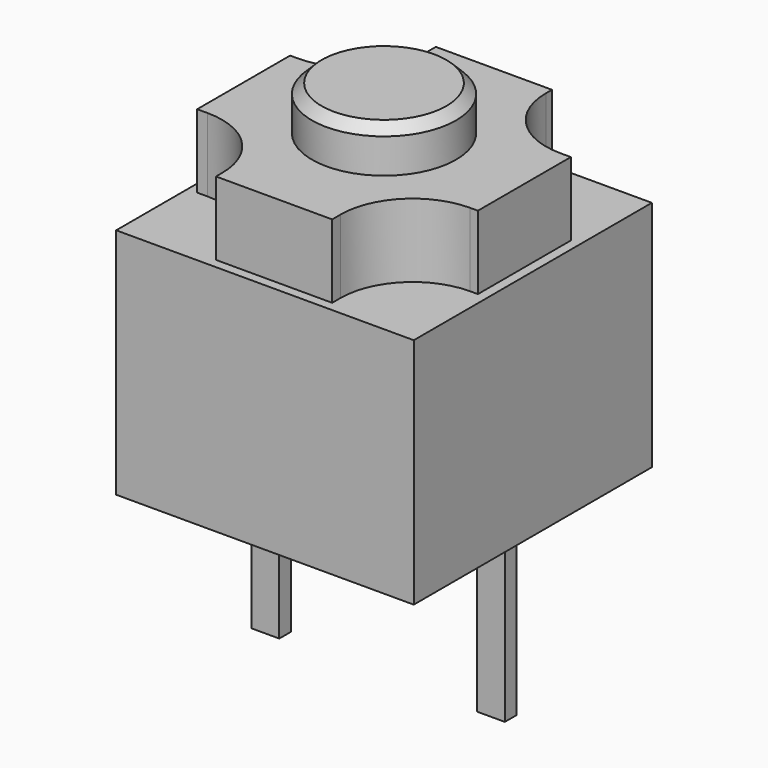
from build123d import *

# Parameters (mm, degrees)
F0_W            = 6.2
F0_H            = 6.2
F1_DEPTH        = 4.85
F3_DEPTH        = 1.53
F3_COPIES_COUNT = 4
F5_R            = 1.5
F6_DEPTH        = 0.92
F7_SIZE         = 0.2
F8_W            = 0.5751895329
F8_H            = 3.9063365496
F9_DEPTH        = 0.15


# Not quite as in the source:
# - a pattern or mirror of a feature is missing from the dataset's text; its kind, count and spacing are read off the source's solid


with BuildPart() as f1:
    # F0 (on Top) → F1 (new body)
    with BuildSketch(Plane.XY):
        Rectangle(F0_W, F0_H)
    extrude(amount=F1_DEPTH)

    # F2 (on face) → F3 (join)
    with BuildSketch(Plane.XY.offset(4.85)):
        with BuildLine():
            Line((1.1802440276, 2.9), (0, 2.9))
            Line((0, 2.9), (0, 0))
            Line((0, 0), (2.9, 0))
            Line((2.9, 0), (2.9, 1.2403748352))
            Line((2.9, 1.2403748352), (2.6802440276, 1.2403748352))
            ThreePointArc((2.6802440276, 1.2403748352), (1.6195838559, 1.6797146634), (1.1802440276, 2.7403748352))
            Line((1.1802440276, 2.7403748352), (1.1802440276, 2.9))
        make_face()
    f3 = extrude(amount=F3_DEPTH)

    # F3_copies: F3 ×4 about axis
    f3_copies_axis = Axis((0, 0, 0), (0, 0, 1))
    for i in range(1, F3_COPIES_COUNT):
        add(f3.rotate(f3_copies_axis, i * 360 / F3_COPIES_COUNT))

    # F5 (on face) → F6 (join)
    with BuildSketch(Plane.XY.offset(6.38)):
        Circle(F5_R)
    extrude(amount=F6_DEPTH)

    # F7
    f7_edges = [f1.edges().sort_by_distance(p)[0] for p in [
        (-1.5, 0, 7.3),
    ]]
    chamfer(f7_edges, length=F7_SIZE)

    # F8 (on Front) → F9 (join, symmetric)
    with BuildSketch(Plane.XZ):
        with Locations((2.35, -1.5468317252)):
            Rectangle(F8_W, F8_H)
    f9 = extrude(amount=F9_DEPTH, both=True)

    # F9_copies: F9 across plane
    add(f9.mirror(Plane(origin=(0, 0, 0), x_dir=(0, 0, -1), z_dir=(-1, 0, 0))))


solid = f1.part
